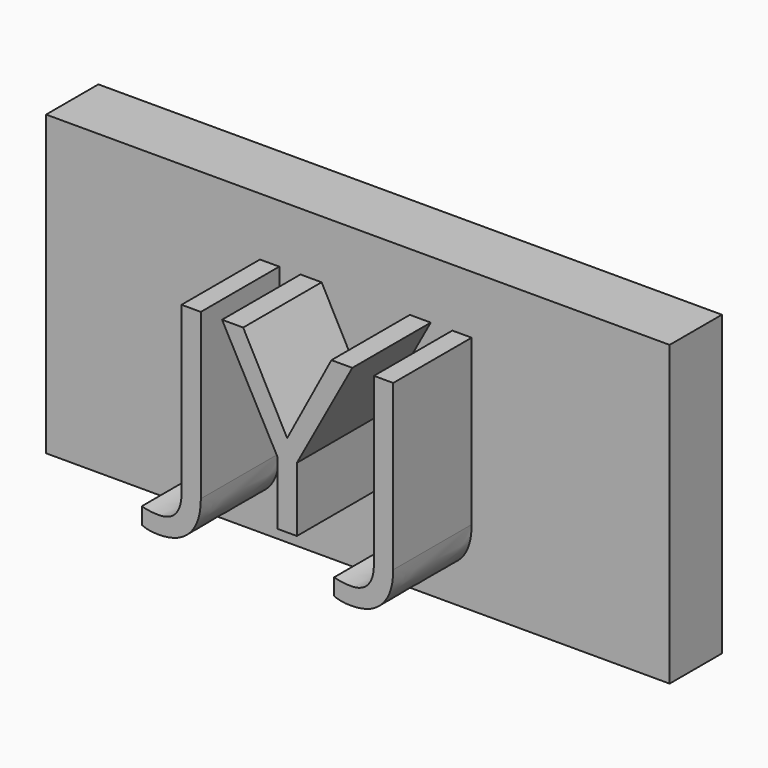
from build123d import *

# Parameters (mm, degrees)
F0_W         = 95.4036265612
F0_H         = 45.6278249621
F1_DEPTH     = 10
F2_TEXT_SIZE = 35.5907276066
F3_DEPTH     = 15


# Not quite as in the source:
# - Text() gives the source's letters only with a copy of the font that has no kerning and outlines rounded to 1/6400 em; it was checked with that copy


with BuildPart() as f1:
    # F0 (on Front) → F1 (new body)
    with BuildSketch(Plane.XZ):
        with Locations((47.7018132806, 22.8139124811)):
            Rectangle(F0_W, F0_H)
    extrude(amount=F1_DEPTH)

    # F2 (on face) → F3 (join)
    with BuildSketch(Plane.XZ.offset(10)):
        with Locations((29.41997163, 11.3378260285)):
            Text('JYJ', F2_TEXT_SIZE, font='Open Sans', text_align=(TextAlign.LEFT, TextAlign.BOTTOM))
    extrude(amount=F3_DEPTH)


solid = f1.part
